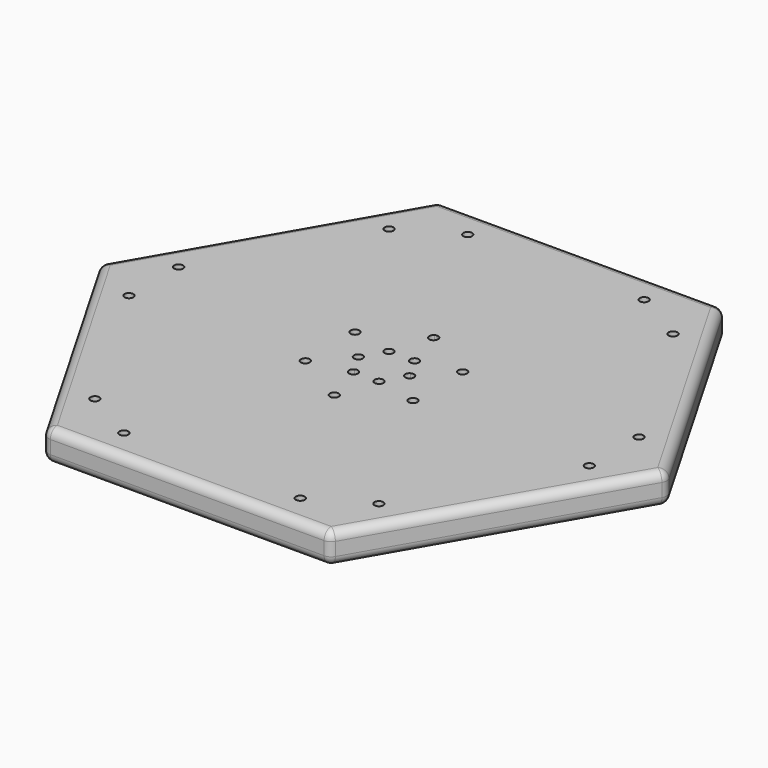
from build123d import *

# Parameters (mm, degrees)
F0_R     = 1
F1_DEPTH = 7
F2_T     = -2.5
F3_R     = 2
F5_DEPTH = 25
F6_DEPTH = 25


with BuildPart() as f1:
    # F0 (on Top) → F1 (new body)
    with BuildSketch(Plane.XY):
        Polygon((0, 0), (-32.0025254212, 55.43), (-64.0050508424, 0), (-32.0025254212, -55.43), (32.0025254212, -55.43), (64.0050508424, 0), (32.0025254212, 55.43), align=None)
        with Locations((-32.0025254212, -41.43)):
            Circle(F0_R, mode=Mode.SUBTRACT)
        with Locations((-19.8781697682, -48.43)):
            Circle(F0_R, mode=Mode.SUBTRACT)
        with Locations((-51.8806951894, -7)):
            Circle(F0_R, mode=Mode.SUBTRACT)
        with Locations((-12.124355653, -7)):
            Circle(F0_R, mode=Mode.SUBTRACT)
        with Locations((19.8781697682, -48.43)):
            Circle(F0_R, mode=Mode.SUBTRACT)
        with Locations((32.0025254212, -41.43)):
            Circle(F0_R, mode=Mode.SUBTRACT)
        with Locations((0, -14)):
            Circle(F0_R, mode=Mode.SUBTRACT)
        with Locations((12.124355653, -7)):
            Circle(F0_R, mode=Mode.SUBTRACT)
        with Locations((51.8806951894, -7)):
            Circle(F0_R, mode=Mode.SUBTRACT)
        with Locations((-51.8806951894, 7)):
            Circle(F0_R, mode=Mode.SUBTRACT)
        with Locations((-12.124355653, 7)):
            Circle(F0_R, mode=Mode.SUBTRACT)
        with Locations((-32.0025254212, 41.43)):
            Circle(F0_R, mode=Mode.SUBTRACT)
        with Locations((12.124355653, 7)):
            Circle(F0_R, mode=Mode.SUBTRACT)
        with Locations((51.8806951894, 7)):
            Circle(F0_R, mode=Mode.SUBTRACT)
        with Locations((32.0025254212, 41.43)):
            Circle(F0_R, mode=Mode.SUBTRACT)
        with BuildLine():
            Line((0, 55.43), (-32.0025254212, 55.43))
            Line((-32.0025254212, 55.43), (0, 0))
            Line((0, 0), (0, 13))
            ThreePointArc((0, 13), (-0.9659258263, 13.7411809549), (-0.5, 14.8660254038))
            Line((-0.5, 14.8660254038), (-19.3781697682, 47.5639745962))
            ThreePointArc((-19.3781697682, 47.5639745962), (-20.744195172, 48.93), (-18.8781697682, 48.43))
            Line((-18.8781697682, 48.43), (0, 48.43))
            Line((0, 48.43), (0, 55.43))
        make_face()
        with BuildLine():
            Line((32.0025254212, 55.43), (0, 55.43))
            Line((0, 55.43), (0, 48.43))
            Line((0, 48.43), (18.8781697682, 48.43))
            ThreePointArc((18.8781697682, 48.43), (19.8781697682, 49.43), (20.8781697682, 48.43))
            ThreePointArc((20.8781697682, 48.43), (20.3781697682, 47.5639745962), (19.3781697682, 47.5639745962))
            Line((19.3781697682, 47.5639745962), (0.5, 14.8660254038))
            ThreePointArc((0.5, 14.8660254038), (0.8660254038, 14.5), (1, 14))
            ThreePointArc((1, 14), (0.7071067812, 13.2928932188), (0, 13))
            Line((0, 13), (0, 0))
            Line((0, 0), (32.0025254212, 55.43))
        make_face()
        with BuildLine():
            Line((0, 15), (0, 48.43))
            Line((0, 48.43), (-18.8781697682, 48.43))
            ThreePointArc((-18.8781697682, 48.43), (-19.0121443644, 47.93), (-19.3781697682, 47.5639745962))
            Line((-19.3781697682, 47.5639745962), (-0.5, 14.8660254038))
            ThreePointArc((-0.5, 14.8660254038), (-0.2588190451, 14.9659258263), (0, 15))
        make_face()
        with BuildLine():
            Line((18.8781697682, 48.43), (0, 48.43))
            Line((0, 48.43), (0, 15))
            ThreePointArc((0, 15), (0.2588190451, 14.9659258263), (0.5, 14.8660254038))
            Line((0.5, 14.8660254038), (19.3781697682, 47.5639745962))
            ThreePointArc((19.3781697682, 47.5639745962), (19.0121443644, 47.93), (18.8781697682, 48.43))
        make_face()
    extrude(amount=F1_DEPTH)

    # F2
    f2_openings = [f1.faces().sort_by_distance(p)[0] for p in [
        (0, 0, 0),
    ]]
    offset(amount=F2_T, openings=f2_openings)

    # F3
    f3_edges = [f1.edges().sort_by_distance(p)[0] for p in [
        (0, -55.43, 7),
        (-48.003788, -27.715, 7),
        (-48.003788, 27.715, 7),
        (0, 55.43, 7),
        (48.003788, 27.715, 7),
        (48.003788, -27.715, 7),
        (48.003788, -27.715, 0),
        (0, -55.43, 0),
        (32.002525, -55.43, 3.5),
        (64.005051, 0, 3.5),
        (48.003788, 27.715, 0),
        (32.002525, 55.43, 3.5),
        (0, 55.43, 0),
        (-32.002525, 55.43, 3.5),
        (-48.003788, 27.715, 0),
        (-64.005051, 0, 3.5),
        (-48.003788, -27.715, 0),
        (-32.002525, -55.43, 3.5),
    ]]
    fillet(f3_edges, radius=F3_R)

    # F4 (on face) → F5 (cut)
    with BuildSketch(Plane.XY.offset(7)):
        with BuildLine():
            Line((-1.8867513459, 5), (-2.8867513459, 5))
            Line((-2.8867513459, 5), (-3.3867513459, 4.1339745962))
            ThreePointArc((-3.3867513459, 4.1339745962), (-2.3867513459, 4.1339745962), (-1.8867513459, 5))
        make_face()
        with BuildLine():
            Line((-3.3867513459, 4.1339745962), (-2.8867513459, 5))
            Line((-2.8867513459, 5), (-1.8867513459, 5))
            ThreePointArc((-1.8867513459, 5), (-3.3867513459, 5.8660254038), (-3.3867513459, 4.1339745962))
        make_face()
    extrude(amount=-F5_DEPTH, mode=Mode.SUBTRACT)

    # F4 (on face) → F6 (cut)
    with BuildSketch(Plane.XY.offset(7)):
        with BuildLine():
            Line((-3.3867513459, 4.1339745962), (-2.8867513459, 5))
            Line((-2.8867513459, 5), (-1.8867513459, 5))
            ThreePointArc((-1.8867513459, 5), (-3.3867513459, 5.8660254038), (-3.3867513459, 4.1339745962))
        make_face()
        with BuildLine():
            Line((-1.8867513459, 5), (-2.8867513459, 5))
            Line((-2.8867513459, 5), (-3.3867513459, 4.1339745962))
            ThreePointArc((-3.3867513459, 4.1339745962), (-2.3867513459, 4.1339745962), (-1.8867513459, 5))
        make_face()
        with BuildLine():
            Line((-5.7735026919, 0), (-5.2735026919, 0.8660254038))
            ThreePointArc((-5.2735026919, 0.8660254038), (-6.7735026919, 0), (-5.2735026919, -0.8660254038))
            Line((-5.2735026919, -0.8660254038), (-5.7735026919, 0))
        make_face()
        with BuildLine():
            ThreePointArc((-4.7735026919, 0), (-4.9074772881, 0.5), (-5.2735026919, 0.8660254038))
            Line((-5.2735026919, 0.8660254038), (-5.7735026919, 0))
            Line((-5.7735026919, 0), (-5.2735026919, -0.8660254038))
            ThreePointArc((-5.2735026919, -0.8660254038), (-4.9074772881, -0.5), (-4.7735026919, 0))
        make_face()
        with BuildLine():
            Line((-2.8867513459, -5), (-3.3867513459, -4.1339745962))
            ThreePointArc((-3.3867513459, -4.1339745962), (-3.3867513459, -5.8660254038), (-1.8867513459, -5))
            Line((-1.8867513459, -5), (-2.8867513459, -5))
        make_face()
        with BuildLine():
            ThreePointArc((-1.8867513459, -5), (-2.3867513459, -4.1339745962), (-3.3867513459, -4.1339745962))
            Line((-3.3867513459, -4.1339745962), (-2.8867513459, -5))
            Line((-2.8867513459, -5), (-1.8867513459, -5))
        make_face()
        with BuildLine():
            ThreePointArc((3.8867513459, -5), (3.7527767497, -4.5), (3.3867513459, -4.1339745962))
            Line((3.3867513459, -4.1339745962), (2.8867513459, -5))
            Line((2.8867513459, -5), (1.8867513459, -5))
            ThreePointArc((1.8867513459, -5), (2.8867513459, -6), (3.8867513459, -5))
        make_face()
        with BuildLine():
            Line((2.8867513459, -5), (3.3867513459, -4.1339745962))
            ThreePointArc((3.3867513459, -4.1339745962), (2.3867513459, -4.1339745962), (1.8867513459, -5))
            Line((1.8867513459, -5), (2.8867513459, -5))
        make_face()
        with BuildLine():
            ThreePointArc((6.7735026919, 0), (6.2735026919, 0.8660254038), (5.2735026919, 0.8660254038))
            Line((5.2735026919, 0.8660254038), (5.7735026919, 0))
            Line((5.7735026919, 0), (5.2735026919, -0.8660254038))
            ThreePointArc((5.2735026919, -0.8660254038), (6.2735026919, -0.8660254038), (6.7735026919, 0))
        make_face()
        with BuildLine():
            Line((5.7735026919, 0), (5.2735026919, 0.8660254038))
            ThreePointArc((5.2735026919, 0.8660254038), (4.7735026919, 0), (5.2735026919, -0.8660254038))
            Line((5.2735026919, -0.8660254038), (5.7735026919, 0))
        make_face()
        with BuildLine():
            Line((2.8867513459, 5), (1.8867513459, 5))
            ThreePointArc((1.8867513459, 5), (2.3867513459, 4.1339745962), (3.3867513459, 4.1339745962))
            Line((3.3867513459, 4.1339745962), (2.8867513459, 5))
        make_face()
        with BuildLine():
            ThreePointArc((3.8867513459, 5), (2.8867513459, 6), (1.8867513459, 5))
            Line((1.8867513459, 5), (2.8867513459, 5))
            Line((2.8867513459, 5), (3.3867513459, 4.1339745962))
            ThreePointArc((3.3867513459, 4.1339745962), (3.7527767497, 4.5), (3.8867513459, 5))
        make_face()
    extrude(amount=-F6_DEPTH, mode=Mode.SUBTRACT)


solid = f1.part
